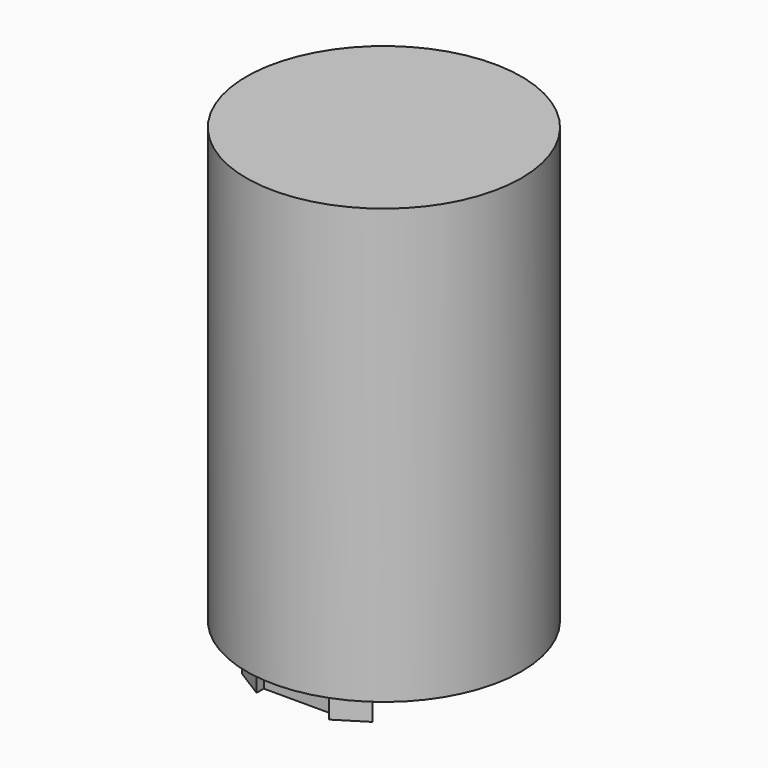
from build123d import *

# Parameters (mm, degrees)
F1_DEPTH = 2
F0_R     = 9.5
F2_DEPTH = 30


with BuildPart() as f1:
    # F0 (on Top) → F1 (new body)
    with BuildSketch(Plane.XY):
        with BuildLine():
            Line((-2.5, -4.5), (-1.25, -4.5))
            Line((-1.25, -4.5), (-1.25, 8))
            ThreePointArc((-1.25, 8), (-1.6246096615, 8.4544378581), (-2.1421771094, 8.1734216623))
            Line((-2.1421771094, 8.1734216623), (-7.2625718321, -4.5))
            Line((-7.2625718321, -4.5), (-6.0125718321, -4.5))
            Line((-6.0125718321, -4.5), (-5.0025062675, -2))
            Line((-5.0025062675, -2), (-2.5, -2))
            Line((-2.5, -2), (-2.5, -4.5))
        make_face()
        Polygon((-2.5, -0.75), (-4.4974734852, -0.75), (-2.5, 4.1939203632), align=None, mode=Mode.SUBTRACT)
    extrude(amount=-F1_DEPTH)


with BuildPart() as f1b:
    # F0 (on Top) → F1, piece 2 (new body)
    with BuildSketch(Plane.XY):
        with BuildLine():
            Line((1.25, 8.4544378581), (1.25, -4.5))
            ThreePointArc((1.25, -4.5), (5.067050605, -1.9109756291), (6.75, 2.3832767911))
            ThreePointArc((6.75, 2.3832767911), (4.9037938648, 6.237624312), (1.25, 8.4544378581))
        make_face()
        Polygon((2.5, -2.2643063941), (2.5, 6.5785330377), (5.502712767, 2.4655844973), align=None, mode=Mode.SUBTRACT)
    extrude(amount=-F1_DEPTH)


with BuildPart() as f1c:
    # F0 (on Top) → F1, piece 3 (new body)
    with BuildSketch(Plane.XY):
        Polygon((2.5, -6), (-2.5, -6), (-2.5, -5.375), (-4.5, -6.625), (-2.5, -7.875), (-2.5, -7.25), (2.5, -7.25), (2.5, -7.875), (4.5, -6.625), (2.5, -5.375), align=None)
    extrude(amount=-F1_DEPTH)


with BuildPart() as f2:
    # F0 (on Top) → F2 (new body)
    with BuildSketch(Plane.XY):
        Circle(F0_R)
        Polygon((-2.5, -5.375), (-2.5, -6), (2.5, -6), (2.5, -5.375), (4.5, -6.625), (2.5, -7.875), (2.5, -7.25), (-2.5, -7.25), (-2.5, -7.875), (-4.5, -6.625), align=None, mode=Mode.SUBTRACT)
        with BuildLine():
            Line((-1.25, 8), (-1.25, -4.5))
            Line((-1.25, -4.5), (-2.5, -4.5))
            Line((-2.5, -4.5), (-2.5, -2))
            Line((-2.5, -2), (-5.0025062675, -2))
            Line((-5.0025062675, -2), (-6.0125718321, -4.5))
            Line((-6.0125718321, -4.5), (-7.2625718321, -4.5))
            Line((-7.2625718321, -4.5), (-2.1421771094, 8.1734216623))
            ThreePointArc((-2.1421771094, 8.1734216623), (-1.6246096615, 8.4544378581), (-1.25, 8))
        make_face(mode=Mode.SUBTRACT)
        with BuildLine():
            ThreePointArc((6.75, 2.3832767911), (5.067050605, -1.9109756291), (1.25, -4.5))
            Line((1.25, -4.5), (1.25, 8.4544378581))
            ThreePointArc((1.25, 8.4544378581), (4.9037938648, 6.237624312), (6.75, 2.3832767911))
        make_face(mode=Mode.SUBTRACT)
        with BuildLine():
            Line((1.25, 8.4544378581), (1.25, -4.5))
            ThreePointArc((1.25, -4.5), (5.067050605, -1.9109756291), (6.75, 2.3832767911))
            ThreePointArc((6.75, 2.3832767911), (4.9037938648, 6.237624312), (1.25, 8.4544378581))
        make_face()
        Polygon((2.5, -2.2643063941), (2.5, 6.5785330377), (5.502712767, 2.4655844973), align=None, mode=Mode.SUBTRACT)
        with BuildLine():
            Line((-2.5, -4.5), (-1.25, -4.5))
            Line((-1.25, -4.5), (-1.25, 8))
            ThreePointArc((-1.25, 8), (-1.6246096615, 8.4544378581), (-2.1421771094, 8.1734216623))
            Line((-2.1421771094, 8.1734216623), (-7.2625718321, -4.5))
            Line((-7.2625718321, -4.5), (-6.0125718321, -4.5))
            Line((-6.0125718321, -4.5), (-5.0025062675, -2))
            Line((-5.0025062675, -2), (-2.5, -2))
            Line((-2.5, -2), (-2.5, -4.5))
        make_face()
        Polygon((-2.5, -0.75), (-4.4974734852, -0.75), (-2.5, 4.1939203632), align=None, mode=Mode.SUBTRACT)
        Polygon((5.502712767, 2.4655844973), (2.5, 6.5785330377), (2.5, -2.2643063941), align=None)
        Polygon((2.5, -6), (-2.5, -6), (-2.5, -5.375), (-4.5, -6.625), (-2.5, -7.875), (-2.5, -7.25), (2.5, -7.25), (2.5, -7.875), (4.5, -6.625), (2.5, -5.375), align=None)
        Polygon((-2.5, 4.1939203632), (-4.4974734852, -0.75), (-2.5, -0.75), align=None)
    extrude(amount=F2_DEPTH)


solid = Compound([f1.part, f1b.part, f1c.part, f2.part])
